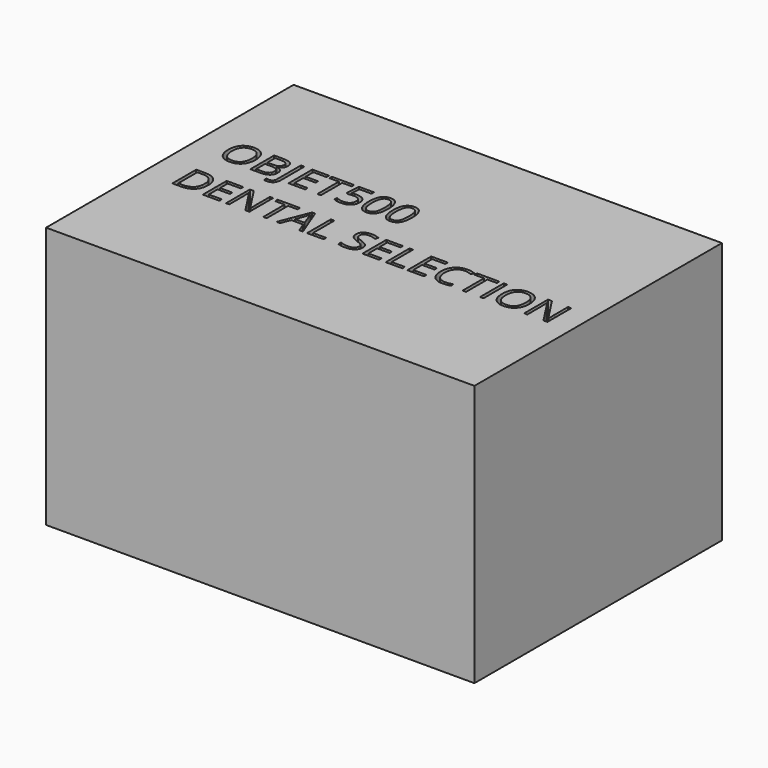
from build123d import *

# Parameters (mm, degrees)
F0_W         = 1800
F0_H         = 1300
F1_DEPTH     = 1100
F2_TEXT_SIZE = 175.4333481253
F3_DEPTH     = 240


# Not quite as in the source:
# - Text() gives the source's letters only with a copy of the font that has no kerning and outlines rounded to 1/6400 em; it was checked with that copy


with BuildPart() as f1:
    # F0 (on Top) → F1 (new body)
    with BuildSketch(Plane.XY):
        Rectangle(F0_W, F0_H)
    extrude(amount=F1_DEPTH)

    # F2 (on face) → F3 (cut)
    with BuildSketch(Plane.XY.offset(1100)):
        with Locations((-790, 93.0125270336)):
            Text('OBJET500', F2_TEXT_SIZE, font='Open Sans', text_align=(TextAlign.LEFT, TextAlign.BOTTOM))
        with Locations((-790, -145.5768264168)):
            Text('DENTAL SELECTION', F2_TEXT_SIZE, font='Open Sans', text_align=(TextAlign.LEFT, TextAlign.BOTTOM))
    extrude(amount=-F3_DEPTH, mode=Mode.SUBTRACT)


solid = f1.part
